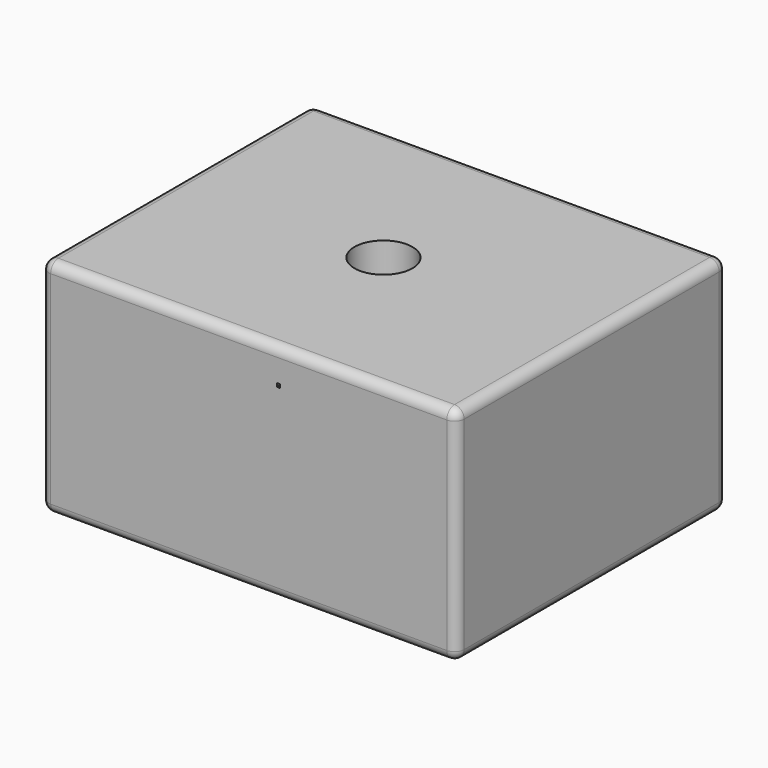
from build123d import *

# Parameters (mm, degrees)
F0_W      = 40
F0_H      = 23
F0_W_2    = 0.3508773884
F0_H_2    = 0.3508765315
F1_DEPTH  = 35
F2_DEPTH  = 3
F3_R      = 1
F4_R      = 1
F8_DEPTH  = 6
F10_R     = 3
F11_DEPTH = 17


# Not quite as in the source:
# - two fillets or chamfers of one size are made in one step


with BuildPart() as f1:
    # F0 (on Front) → F1 (new body)
    with BuildSketch(Plane.XZ):
        with Locations((-11.8218250573, 18.8361621085)):
            Rectangle(F0_W, F0_H)
        with Locations((-10.2428785232, 26.8098455974)):
            Rectangle(F0_W_2, F0_H_2, mode=Mode.SUBTRACT)
    extrude(amount=F1_DEPTH)

    # F2 (add): a face of the model
    f2_faces = [f1.faces().sort_by_distance(p)[0] for p in [
        (-31.8218250573, -17.5, 18.8361621085),
    ]]
    extrude(f2_faces, amount=F2_DEPTH)

    # F3
    f3_edges = [f1.edges().sort_by_distance(p)[0] for p in [
        (-13.321825, -35, 30.336162),
    ]]
    fillet(f3_edges, radius=F3_R)

    # F4
    f4_edges = [f1.edges().sort_by_distance(p)[0] for p in [
        (-13.321825, -35, 7.336162),
        (8.178175, -17, 30.336162),
        (8.178175, -17.5, 7.336162),
        (-13.321825, 0, 30.336162),
        (-13.321825, 0, 7.336162),
        (-34.821825, -17, 30.336162),
        (8.178175, -34.707107, 30.043269),
        (8.178175, 0, 18.836162),
        (8.178175, -35, 18.336162),
        (-34.821825, -34.707107, 30.043269),
        (-34.821825, 0, 18.836162),
        (-34.821825, -35, 18.336162),
        (-34.821825, -17.5, 7.336162),
    ]]
    fillet(f4_edges, radius=F4_R)

    # F7 (on face) → F8 (cut)
    with BuildSketch(Plane(origin=(0, 0, 7.3361621085), x_dir=(1, 0, 0), z_dir=(0, 0, -1))):
        Polygon((-15.4886602973, 23.0950714957), (-19.2507167286, 18.4210013842), (-17.0838814885, 12.8259298884), (-11.1549898172, 11.9049285043), (-7.3929333859, 16.5789986158), (-9.559768626, 22.1740701116), align=None)
    extrude(amount=-F8_DEPTH, mode=Mode.SUBTRACT)

    # F10 (on face) → F11 (cut, through all)
    with BuildSketch(Plane(origin=(0, 0, 13.3361621085), x_dir=(1, 0, 0), z_dir=(0, 0, -1))):
        with Locations((-13.3786574006, 17.5000000745)):
            Circle(F10_R)
    extrude(amount=-F11_DEPTH, mode=Mode.SUBTRACT)


solid = f1.part
